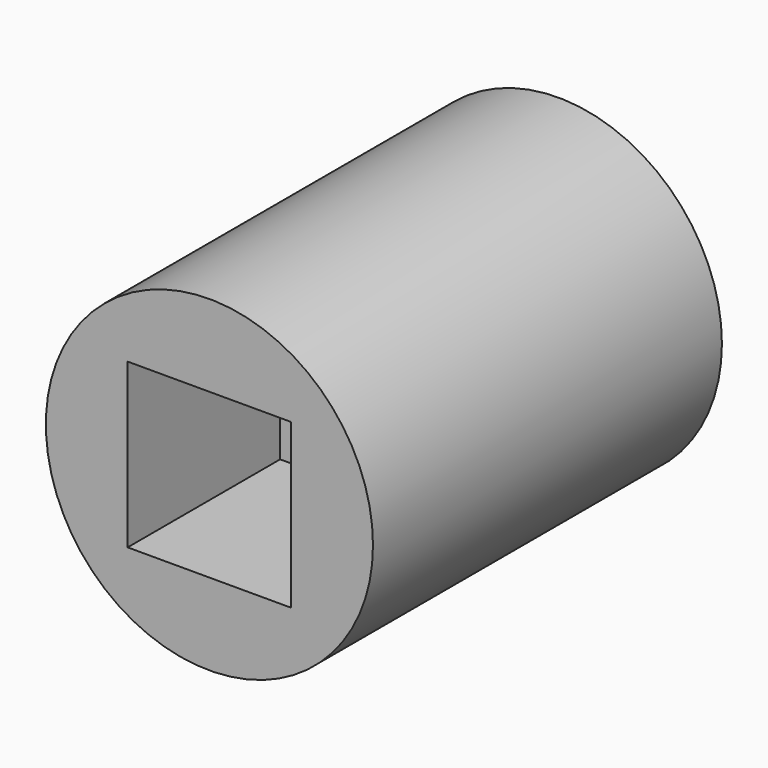
from build123d import *

# Parameters (mm, degrees)
F0_R          = 9.525
F1_DEPTH      = 25.4
F3_DEPTH      = 25.4
F3_DEPTH_BACK = 50
F4_DEPTH      = 11.0998
F7_DEPTH      = 9.525


# Not quite as in the source:
# - an extrude ends at something that could not be found from the text; its depth is read off the source's solid


with BuildPart() as f1:
    # F0 (on Front) → F1 (new body)
    with BuildSketch(Plane.XZ):
        Circle(F0_R)
    extrude(amount=F1_DEPTH)

    # F2 (on face) → F3 (cut, two sides)
    with BuildSketch(Plane.XZ.offset(25.4)) as f3_sk:
        with BuildLine():
            ThreePointArc((4.7625, 0), (3.3675960454, 3.3675960454), (0, 4.7625))
            ThreePointArc((0, 4.7625), (-3.3675960454, 3.3675960454), (-4.7625, 0))
            ThreePointArc((-4.7625, 0), (-3.3675960454, -3.3675960454), (0, -4.7625))
            ThreePointArc((0, -4.7625), (3.3675960454, -3.3675960454), (4.7625, 0))
        make_face()
    extrude(amount=-F3_DEPTH, mode=Mode.SUBTRACT)
    extrude(f3_sk.sketch, amount=F3_DEPTH_BACK, mode=Mode.SUBTRACT)

    # F2 (on face) → F4 (cut)
    with BuildSketch(Plane.XZ.offset(25.4)):
        with BuildLine():
            Line((0, 4.7625), (-4.7625, 4.7625))
            Line((-4.7625, 4.7625), (-4.7625, 0))
            ThreePointArc((-4.7625, 0), (-3.3675960454, 3.3675960454), (0, 4.7625))
        make_face()
        with BuildLine():
            Line((4.7625, 4.7625), (0, 4.7625))
            ThreePointArc((0, 4.7625), (3.3675960454, 3.3675960454), (4.7625, 0))
            Line((4.7625, 0), (4.7625, 4.7625))
        make_face()
        with BuildLine():
            ThreePointArc((4.7625, 0), (3.3675960454, 3.3675960454), (0, 4.7625))
            ThreePointArc((0, 4.7625), (-3.3675960454, 3.3675960454), (-4.7625, 0))
            ThreePointArc((-4.7625, 0), (-3.3675960454, -3.3675960454), (0, -4.7625))
            ThreePointArc((0, -4.7625), (3.3675960454, -3.3675960454), (4.7625, 0))
        make_face()
        with BuildLine():
            ThreePointArc((0, -4.7625), (-3.3675960454, -3.3675960454), (-4.7625, 0))
            Line((-4.7625, 0), (-4.7625, -4.7625))
            Line((-4.7625, -4.7625), (0, -4.7625))
        make_face()
        with BuildLine():
            Line((4.7625, -4.7625), (4.7625, 0))
            ThreePointArc((4.7625, 0), (3.3675960454, -3.3675960454), (0, -4.7625))
            Line((0, -4.7625), (4.7625, -4.7625))
        make_face()
    extrude(amount=-F4_DEPTH, mode=Mode.SUBTRACT)

    # F6 (on face) → F7 (cut)
    with BuildSketch(Plane(origin=(0, 0, 0), x_dir=(-1, 0, 0), z_dir=(0, 1, 0))):
        Polygon((3.6155293455, -6.3447738406), (7.3025, -0.041246659), (3.6869706545, 6.3035271816), (-3.6155293455, 6.3447738406), (-7.3025, 0.041246659), (-3.6869706545, -6.3035271816), align=None)
    extrude(amount=-F7_DEPTH, mode=Mode.SUBTRACT)


solid = f1.part
